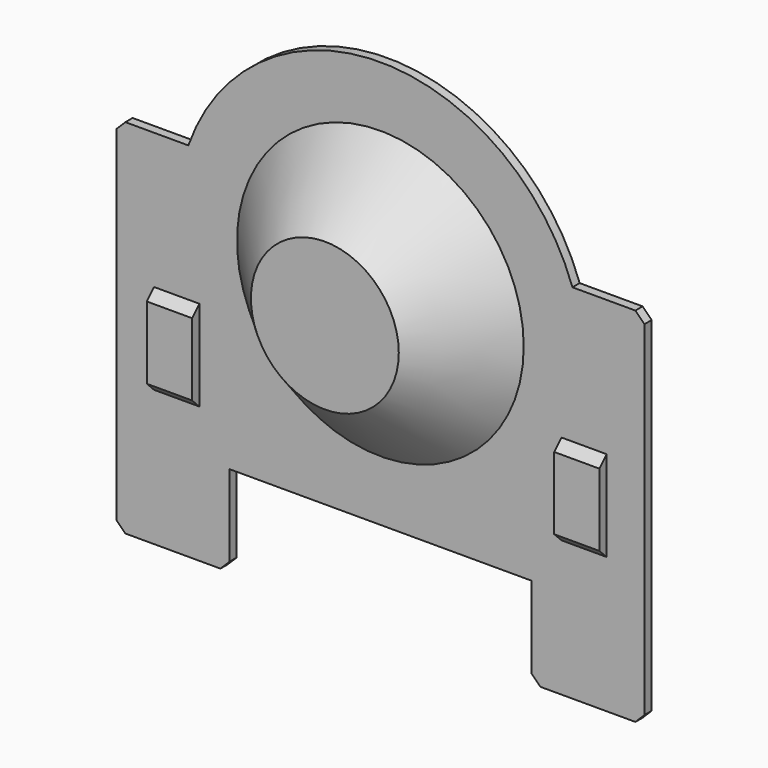
from build123d import *

# Parameters (mm, degrees)
F0_W     = 1.5
F0_H     = 3
F1_DEPTH = 0.3
F2_DEPTH = 0.6
F3_R     = 4.75
F4_DEPTH = 2.3
F5_SIZE  = 2.29999
F6_SIZE  = 0.29999


# Not quite as in the source:
# - a fillet or chamfer is up to 0.001 mm smaller than in the source, because OpenCascade refuses the exact size


with BuildPart() as f1:
    # F0 (on Front) → F1 (new body)
    with BuildSketch(Plane.XZ):
        with BuildLine():
            Line((8.75, -6), (8.75, 6))
            Line((8.75, 6), (6.3639610307, 6))
            ThreePointArc((6.3639610307, 6), (0, 10.5), (-6.3639610307, 6))
            Line((-6.3639610307, 6), (-8.75, 6))
            Line((-8.75, 6), (-8.75, -6))
            Line((-8.75, -6), (-5, -6))
            Line((-5, -6), (-5, -3))
            Line((-5, -3), (5, -3))
            Line((5, -3), (5, -6))
            Line((5, -6), (8.75, -6))
        make_face()
        with Locations((-6.75, 0)):
            Rectangle(F0_W, F0_H, mode=Mode.SUBTRACT)
        with Locations((6.75, 0)):
            Rectangle(F0_W, F0_H, mode=Mode.SUBTRACT)
        with Locations((-6.75, 0)):
            Rectangle(F0_W, F0_H)
        with Locations((6.75, 0)):
            Rectangle(F0_W, F0_H)
    extrude(amount=F1_DEPTH)

    # F0 (on Front) → F2 (join)
    with BuildSketch(Plane.XZ):
        with Locations((-6.75, 0)):
            Rectangle(F0_W, F0_H)
        with Locations((6.75, 0)):
            Rectangle(F0_W, F0_H)
    extrude(amount=F2_DEPTH)

    # F3 (on face) → F4 (join)
    with BuildSketch(Plane.XZ.offset(0.3)):
        with Locations((0, 3.75)):
            Circle(F3_R)
    extrude(amount=F4_DEPTH)

    # F5 (size 2.3 in the source; OpenCascade refuses exactly that, so slightly less here)
    f5_edges = [f1.edges().sort_by_distance(p)[0] for p in [
        (-4.75, -2.6, 3.75),
    ]]
    chamfer(f5_edges, length=F5_SIZE)

    # F6 (size 0.3 in the source; OpenCascade refuses exactly that, so slightly less here)
    f6_edges = [f1.edges().sort_by_distance(p)[0] for p in [
        (-6.75, -0.6, -1.5),
        (-6.75, -0.6, 1.5),
        (6.75, -0.6, -1.5),
        (6.75, -0.6, 1.5),
        (-5, -0.15, -6),
        (-8.75, -0.15, -6),
        (5, -0.15, -6),
        (8.75, -0.15, -6),
        (8.75, -0.15, 6),
        (-8.75, -0.15, 6),
    ]]
    chamfer(f6_edges, length=F6_SIZE)


solid = f1.part
